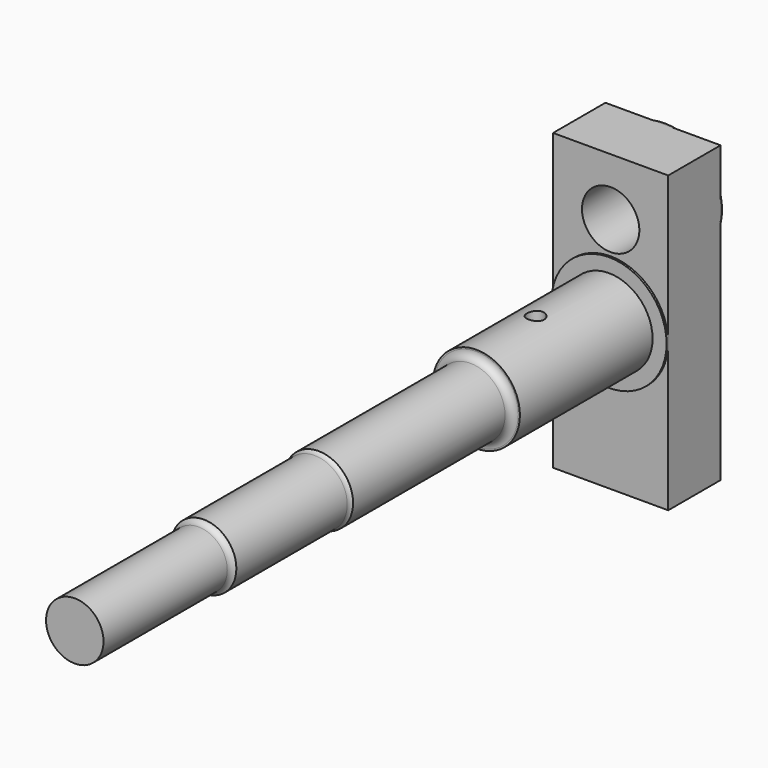
from build123d import *

# Parameters (mm, degrees)
F1_DEPTH  = 9.017
F2_R      = 7.9375
F3_DEPTH  = 0.2794
F4_R      = 6.00075
F5_DEPTH  = 22.86
F6_R      = 4.76123
F7_DEPTH  = 50.0634
F8_R      = 4.49961
F9_DEPTH  = 69.85
F10_R     = 3.9624
F11_DEPTH = 92.075
F15_W     = 1.1811
F15_H     = 2.286
F17_R     = 7.9375
F18_DEPTH = 0.254
F19_R     = 3.95097
F20_DEPTH = 25.4
F21_R     = 1.7526
F22_DEPTH = 9.525


# Not quite as in the source:
# - a fillet or chamfer that OpenCascade refuses, or shapes differently, is made with other operations: its cross-section is extruded or revolved along the edge and cut away or added
# - a feature of the source that left no trace in its solid (it failed there, or was rolled back) is left out


with BuildPart() as f1:
    # F0 (on Front) → F1 (new body)
    with BuildSketch(Plane.XZ):
        Polygon((7.9375, 20.32), (0, 20.32), (-7.9375, 20.32), (-7.9375, 0), (-7.9375, -20.32), (0, -20.32), (7.9375, -20.32), (7.9375, 0), align=None)
    extrude(amount=F1_DEPTH)

    # F2 (on face) → F3 (join)
    with BuildSketch(Plane.XZ.offset(9.017)):
        Circle(F2_R)
    extrude(amount=F3_DEPTH)

    # F4 (on face) → F5 (join)
    with BuildSketch(Plane.XZ.offset(9.2964)):
        Circle(F4_R)
    extrude(amount=F5_DEPTH)

    # F6 (on face) → F7 (join)
    with BuildSketch(Plane.XZ.offset(9.2964)):
        Circle(F6_R)
    extrude(amount=F7_DEPTH)

    # F8 (on face) → F9 (join)
    with BuildSketch(Plane.XZ.offset(9.2964)):
        Circle(F8_R)
    extrude(amount=F9_DEPTH)

    # F10 (on face) → F11 (join)
    with BuildSketch(Plane.XZ.offset(9.2964)):
        Circle(F10_R)
    extrude(amount=F11_DEPTH)

    # F14: fillet of radius 1.016 on 3 edges, made by hand

    # F14_s1 → F14_t2 (revolve)
    with BuildSketch(Plane.XY):
        with BuildLine():
            ThreePointArc((5.77723, -32.1564), (5.0588095103, -32.4539795103), (4.76123, -33.1724))
            Line((4.76123, -33.1724), (4.76123, -32.1564))
            Line((4.76123, -32.1564), (5.77723, -32.1564))
        make_face()
    revolve(axis=Axis((0, -32.1564, 0), (0, 1, 0)))

    # F14_s3 → F14_t4 (revolve)
    with BuildSketch(Plane.XY):
        with BuildLine():
            ThreePointArc((4.76123, -59.3598), (4.5672677411, -59.675805019), (4.49961, -60.0403636014))
            Line((4.49961, -60.0403636014), (4.49961, -59.3598))
            Line((4.49961, -59.3598), (4.76123, -59.3598))
        make_face()
    revolve(axis=Axis((0, -59.3598, 0), (0, 1, 0)))

    # F14_s5 → F14_t6 (revolve)
    with BuildSketch(Plane.XY):
        with BuildLine():
            ThreePointArc((4.49961, -79.1464), (4.1069911866, -79.5201107955), (3.9624, -80.042511676))
            Line((3.9624, -80.042511676), (3.9624, -79.1464))
            Line((3.9624, -79.1464), (4.49961, -79.1464))
        make_face()
    revolve(axis=Axis((0, -79.1464, 0), (0, 1, 0)))

    # F15 (on Right) → F16 (revolve, cut)
    with BuildSketch(Plane.YZ):
        with Locations((-21.38045, 4.85775)):
            Rectangle(F15_W, F15_H)
    revolve(axis=Axis((0, -21.971, 4.85775), (0, 0, -1)), mode=Mode.SUBTRACT)

    # F17 (on face) → F18 (join)
    with BuildSketch(Plane(origin=(0, 0, 0), x_dir=(-1, 0, 0), z_dir=(0, 1, 0))):
        with Locations((0, 12.3825)):
            Circle(F17_R)
    extrude(amount=F18_DEPTH)

    # F19 (on face) → F20 (cut)
    with BuildSketch(Plane(origin=(0, 0.254, 0), x_dir=(-1, 0, 0), z_dir=(0, 1, 0))):
        with Locations((0, 12.3825)):
            Circle(F19_R)
    extrude(amount=-F20_DEPTH, mode=Mode.SUBTRACT)

    # F21 (on face) → F22 (cut)
    with BuildSketch(Plane(origin=(0, 0, -20.32), x_dir=(1, 0, 0), z_dir=(0, 0, -1))):
        with Locations((4.445, 4.5085)):
            Circle(F21_R)
        with Locations((-4.445, 4.5085)):
            Circle(F21_R)
    extrude(amount=-F22_DEPTH, mode=Mode.SUBTRACT)


solid = f1.part
